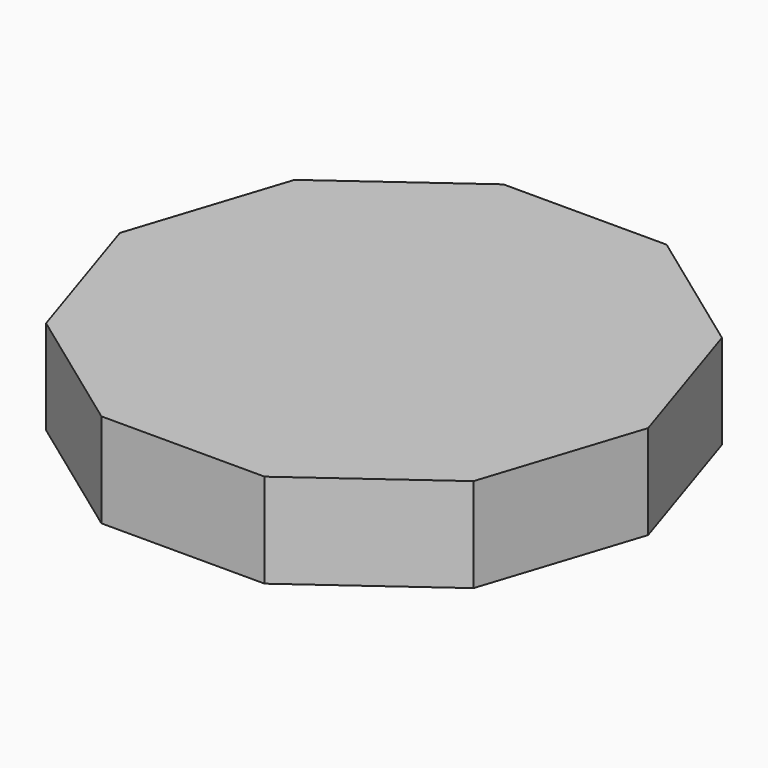
from build123d import *

# Parameters (mm, degrees)
F1_DEPTH = 19.05
F2_W     = 70.8835957375
F2_H     = 27.94
F3_DEPTH = 3.175
F4_R     = 12.6886346665
F5_DEPTH = 14.732


# Not quite as in the source:
# - a fillet or chamfer that OpenCascade refuses, or shapes differently, is made with other operations: its cross-section is extruded or revolved along the edge and cut away or added


with BuildPart() as f1:
    # F0 (on Top) → F1 (new body)
    with BuildSketch(Plane.XY):
        Polygon((-16.5059205686, -50.8), (16.5059205686, -50.8), (43.2130610643, -31.3961266285), (53.4142809913, 0), (43.2130610643, 31.3961266285), (16.5059205686, 50.8), (-16.5059205686, 50.8), (-43.2130610643, 31.3961266285), (-53.4142809913, 0), (-43.2130610643, -31.3961266285), align=None)
    extrude(amount=F1_DEPTH)

    # F2 (on face) → F3 (join)
    with BuildSketch(Plane(origin=(0, 0, 0), x_dir=(1, 0, 0), z_dir=(0, 0, -1))):
        Rectangle(F2_W, F2_H)
    extrude(amount=F3_DEPTH)

    # F4 (on face) → F5 (join)
    with BuildSketch(Plane(origin=(0, 0, -3.175), x_dir=(1, 0, 0), z_dir=(0, 0, -1))):
        Circle(F4_R)
    extrude(amount=F5_DEPTH)

    # F6: chamfer of 12.6873 x 15.1201353553 on 1 edges, made by hand


with BuildPart() as f6_tool2:
    # F6_s3 → F6_t4 (revolve)
    with BuildSketch(Plane.XZ):
        Polygon((12.6886346665, -2.7868646447), (0.0013346665, -17.907), (12.6886346665, -17.907), align=None)
    revolve(axis=Axis((0, 0, -17.907), (0, 0, -1)))

    split(bisect_by=Plane.XY.offset(-3.175), keep=Keep.BOTTOM)


with BuildPart() as f1_1:
    add(f1.part)

    # F6_t1: cut F6_tool2
    add(f6_tool2.part, mode=Mode.SUBTRACT)


solid = f1_1.part
